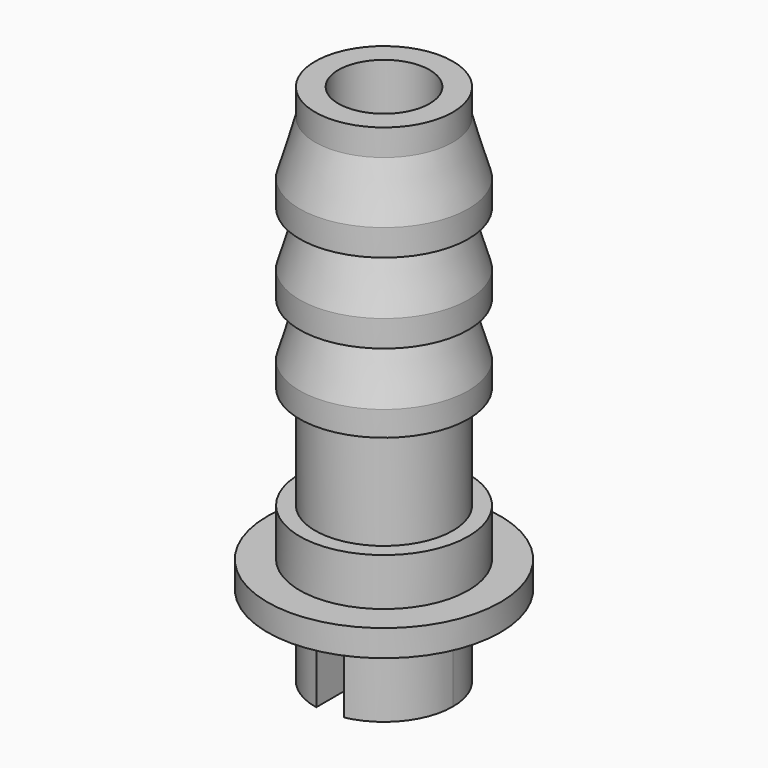
from build123d import *

# Parameters (mm, degrees)
F0_R      = 3.385
F1_DEPTH  = 15.2
F2_R      = 3.385
F3_DEPTH  = 2.35
F4_DEPTH  = 1.65
F6_R      = 3.385
F6_R_2    = 2.45
F7_DEPTH  = 12.08
F9_R      = 3.385
F9_R_2    = 2
F10_DEPTH = 3
F11_R     = 2.45
F11_R_2   = 2
F12_DEPTH = 0.77
F31_R     = 1.325
F32_DEPTH = 13.55


with BuildPart() as f1:
    # F0 (on Top) → F1 (new body)
    with BuildSketch(Plane.XY):
        Circle(F0_R)
    extrude(amount=F1_DEPTH)

    # F2 (on face) → F3 (cut)
    with BuildSketch(Plane(origin=(0, 0, 0), x_dir=(1, 0, 0), z_dir=(0, 0, -1))):
        Circle(F2_R)
        with BuildLine():
            ThreePointArc((0.4, 1.9595917942), (1.5491933385, 1.2649110641), (2, 0))
            ThreePointArc((2, 0), (1.5491933385, -1.2649110641), (0.4, -1.9595917942))
            ThreePointArc((0.4, -1.9595917942), (0, -2), (-0.4, -1.9595917942))
            ThreePointArc((-0.4, -1.9595917942), (-2, 0), (-0.4, 1.9595917942))
            ThreePointArc((-0.4, 1.9595917942), (0, 2), (0.4, 1.9595917942))
        make_face(mode=Mode.SUBTRACT)
    extrude(amount=-F3_DEPTH, mode=Mode.SUBTRACT)

    # F2 (on face) → F4 (cut)
    with BuildSketch(Plane(origin=(0, 0, 0), x_dir=(1, 0, 0), z_dir=(0, 0, -1))):
        with BuildLine():
            Line((0.4, -1.9595917942), (0.4, 1.9595917942))
            ThreePointArc((0.4, 1.9595917942), (0, 2), (-0.4, 1.9595917942))
            Line((-0.4, 1.9595917942), (-0.4, -1.9595917942))
            ThreePointArc((-0.4, -1.9595917942), (0, -2), (0.4, -1.9595917942))
        make_face()
    extrude(amount=-F4_DEPTH, mode=Mode.SUBTRACT)

    # F6 (on face) → F7 (cut, through all)
    with BuildSketch(Plane.XY.offset(15.2)):
        Circle(F6_R)
        Circle(F6_R_2, mode=Mode.SUBTRACT)
    extrude(amount=-F7_DEPTH, mode=Mode.SUBTRACT)

    # F9 (on offset) → F10 (cut)
    with BuildSketch(Plane.XY.offset(4.5)):
        Circle(F9_R)
        Circle(F9_R_2, mode=Mode.SUBTRACT)
    extrude(amount=F10_DEPTH, mode=Mode.SUBTRACT)

    # F11 (on face) → F12 (cut)
    with BuildSketch(Plane.XY.offset(15.2)):
        Circle(F11_R)
        Circle(F11_R_2, mode=Mode.SUBTRACT)
    extrude(amount=-F12_DEPTH, mode=Mode.SUBTRACT)

    # F20 (on Front) → F28 (revolve, cut)
    with BuildSketch(Plane.XZ):
        Polygon((-2.45, 14.43), (-2.45, 12.875), (-2, 14.43), align=None)
    revolve(axis=Axis((0, 0, 10.2299177088), (0, 0, -1)), mode=Mode.SUBTRACT)

    # F23 (on Front) → F29 (revolve, cut)
    with BuildSketch(Plane.XZ):
        Polygon((-2.45, 12.105), (-2.45, 10.55), (-2, 12.105), align=None)
    revolve(axis=Axis((0, 0, 10.2299177088), (0, 0, -1)), mode=Mode.SUBTRACT)

    # F26 (on Front) → F30 (revolve, cut)
    with BuildSketch(Plane.XZ):
        Polygon((-2.45, 9.78), (-2.45, 8.225), (-2, 9.78), align=None)
    revolve(axis=Axis((0, 0, 10.2299177088), (0, 0, -1)), mode=Mode.SUBTRACT)

    # F31 (on face) → F32 (cut, through all)
    with BuildSketch(Plane.XY.offset(15.2)):
        Circle(F31_R)
    extrude(amount=-F32_DEPTH, mode=Mode.SUBTRACT)


solid = f1.part
